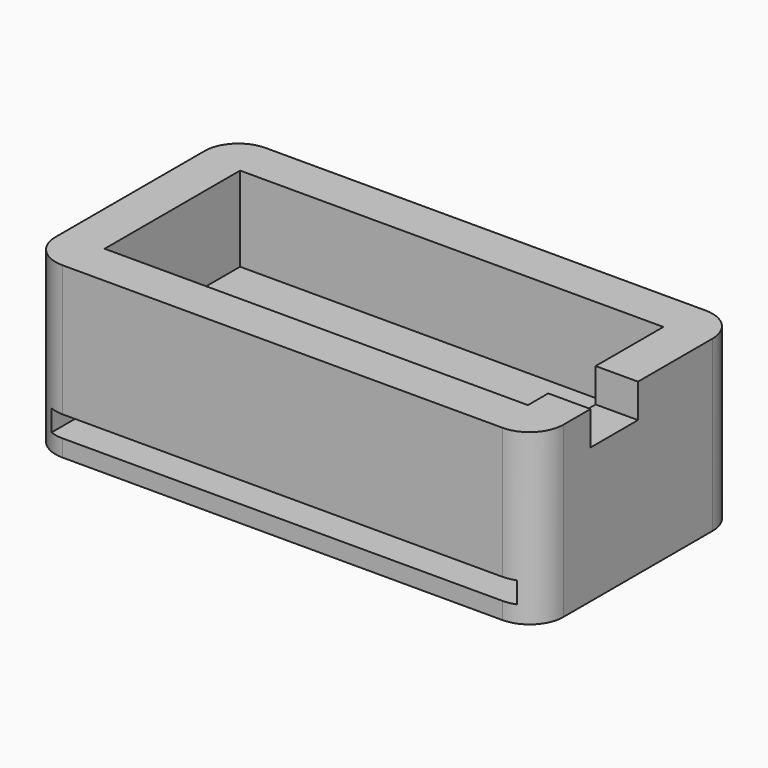
from build123d import *

# Parameters (mm, degrees)
F0_W        = 76.2
F0_H        = 38.1
F1_DEPTH    = 25.4
F2_W        = 69.85
F2_H        = 3.175
F3_DEPTH    = 38.101
F4_W        = 63.5
F4_H        = 25.4
F5_DEPTH    = 12.7
F6_W        = 6.35
F6_H        = 8.89
F7_DEPTH    = 5.08
F8_T1_DEPTH = 50.8


# Not quite as in the source:
# - a fillet or chamfer that OpenCascade refuses, or shapes differently, is made with other operations: its cross-section is extruded or revolved along the edge and cut away or added


with BuildPart() as f1:
    # F0 (on Top) → F1 (new body)
    with BuildSketch(Plane.XY):
        with Locations((6.725884974, -8.772585205)):
            Rectangle(F0_W, F0_H)
    extrude(amount=F1_DEPTH)

    # F2 (on face) → F3 (cut, through all)
    with BuildSketch(Plane.XZ.offset(27.822585205)):
        with Locations((6.725884974, 4.1275)):
            Rectangle(F2_W, F2_H)
    extrude(amount=-F3_DEPTH, mode=Mode.SUBTRACT)

    # F4 (on face) → F5 (cut)
    with BuildSketch(Plane.XY.offset(25.4)):
        with Locations((6.725884974, -8.772585205)):
            Rectangle(F4_W, F4_H)
    extrude(amount=-F5_DEPTH, mode=Mode.SUBTRACT)

    # F6 (on face) → F7 (cut)
    with BuildSketch(Plane.XY.offset(25.4)):
        with Locations((41.650884974, -13.217585205)):
            Rectangle(F6_W, F6_H)
    extrude(amount=-F7_DEPTH, mode=Mode.SUBTRACT)

    # F8: fillet of radius 5.08 on 4 edges, made by hand

    # F8_s2 → F8_t1 (cut)
    with BuildSketch(Plane.XY.offset(-12.7)):
        with BuildLine():
            ThreePointArc((44.825884974, 5.197414795), (43.3379874224, 8.7895172434), (39.745884974, 10.277414795))
            Line((39.745884974, 10.277414795), (44.825884974, 10.277414795))
            Line((44.825884974, 10.277414795), (44.825884974, 5.197414795))
        make_face()
        with BuildLine():
            ThreePointArc((-26.294115026, 10.277414795), (-29.8862174744, 8.7895172434), (-31.374115026, 5.197414795))
            Line((-31.374115026, 5.197414795), (-31.374115026, 10.277414795))
            Line((-31.374115026, 10.277414795), (-26.294115026, 10.277414795))
        make_face()
        with BuildLine():
            ThreePointArc((44.825884974, -22.742585205), (43.3379874224, -26.3346876534), (39.745884974, -27.822585205))
            Line((39.745884974, -27.822585205), (44.825884974, -27.822585205))
            Line((44.825884974, -27.822585205), (44.825884974, -22.742585205))
        make_face()
        with BuildLine():
            ThreePointArc((-26.294115026, -27.822585205), (-29.8862174744, -26.3346876534), (-31.374115026, -22.742585205))
            Line((-31.374115026, -22.742585205), (-31.374115026, -27.822585205))
            Line((-31.374115026, -27.822585205), (-26.294115026, -27.822585205))
        make_face()
    extrude(amount=F8_T1_DEPTH, mode=Mode.SUBTRACT)


solid = f1.part
